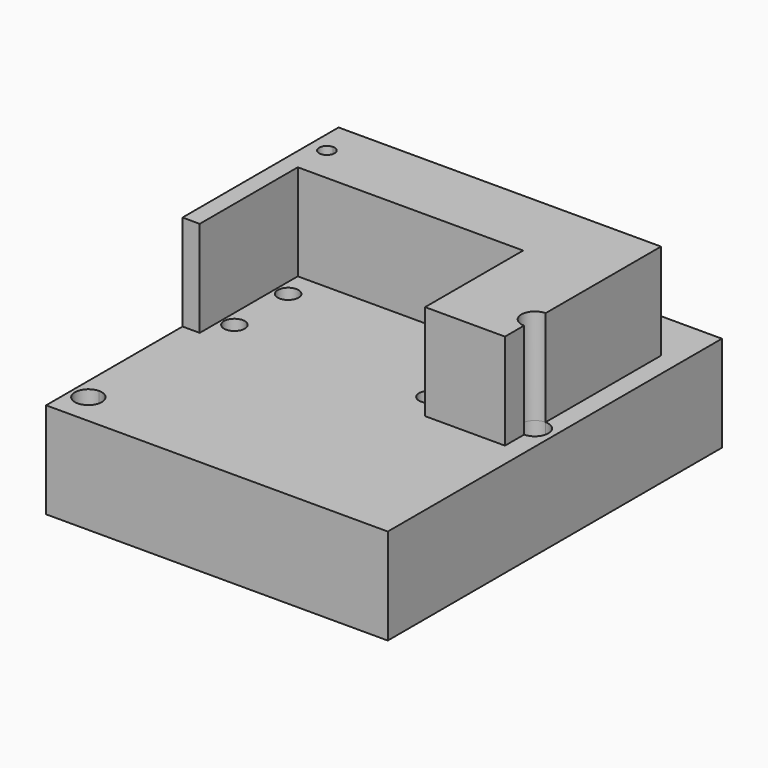
from build123d import *
from build123d import SkipClean  # not in build123d's __all__

# Parameters (mm, degrees)
F0_W     = 58.7
F0_H     = 31.916891567
F0_W_2   = 50.8
F0_H_2   = 17.5
F0_W_3   = 1.3
F0_H_3   = 0.083108433
F1_DEPTH = 25
F2_D     = 5.4102
F3_DEPTH = 25


with BuildPart() as f1:
    # F0 (on Top) → F1 (new body)
    with BuildSketch(Plane.XY):
        with BuildLine():
            ThreePointArc((0, 3.5), (2.4748737342, 2.4748737342), (3.5, 0))
            Line((3.5, 0), (79.5, 0))
            Line((79.5, 0), (79.5, 36.256108433))
            Line((79.5, 36.256108433), (58.7, 36.256108433))
            Line((58.7, 36.256108433), (58.7, 36.173))
            Line((58.7, 36.173), (0, 36.173))
            Line((0, 36.173), (0, 3.5))
        make_face()
        with BuildLine():
            Line((58.7, 36.256108433), (79.5, 36.256108433))
            Line((79.5, 36.256108433), (79.5, 42.475))
            ThreePointArc((79.5, 42.475), (76, 45.975), (79.5, 49.475))
            Line((79.5, 49.475), (79.5, 87.056108433))
            Line((79.5, 87.056108433), (0, 87.056108433))
            Line((0, 87.056108433), (0, 79.6536390185))
            ThreePointArc((0, 79.6536390185), (1.4142135624, 79.0678525809), (2, 77.6536390185))
            ThreePointArc((2, 77.6536390185), (1.4142135624, 76.2394254562), (0, 75.6536390185))
            Line((0, 75.6536390185), (0, 68.173))
            Line((0, 68.173), (58.7, 68.173))
            Line((58.7, 68.173), (58.7, 36.256108433))
        make_face()
        with Locations((29.35, 52.2145542165)):
            Rectangle(F0_W, F0_H)
        with Locations((28.7, 52.173)):
            Rectangle(F0_W_2, F0_H_2, mode=Mode.SUBTRACT)
        with BuildLine():
            Line((79.5, 0), (3.5, 0))
            ThreePointArc((3.5, 0), (-2.4748737342, -2.4748737342), (0, 3.5))
            Line((0, 3.5), (0, 36.173))
            Line((0, 36.173), (-1.3, 36.173))
            Line((-1.3, 36.173), (-1.3, 36.256108433))
            Line((-1.3, 36.256108433), (-4.48, 36.256108433))
            Line((-4.48, 36.256108433), (-4.48, -8.1671467051))
            Line((-4.48, -8.1671467051), (84.52, -8.1671467051))
            Line((84.52, -8.1671467051), (84.52, 36.256108433))
            Line((84.52, 36.256108433), (79.5, 36.256108433))
            Line((79.5, 36.256108433), (79.5, 0))
        make_face()
        with Locations((28.7, 52.173)):
            Rectangle(F0_W_2, F0_H_2)
        with BuildLine():
            Line((79.5, 87.056108433), (84.52, 87.056108433))
            Line((84.52, 87.056108433), (84.52, 100.6101816893))
            Line((84.52, 100.6101816893), (28.7, 100.6101816893))
            Line((28.7, 100.6101816893), (-4.48, 100.6101816893))
            Line((-4.48, 100.6101816893), (-4.48, 87.056108433))
            Line((-4.48, 87.056108433), (0, 87.056108433))
            Line((0, 87.056108433), (0, 88.45))
            ThreePointArc((0, 88.45), (-2.4748737342, 94.4248737342), (3.5, 91.95))
            Line((3.5, 91.95), (79.5, 91.95))
            Line((79.5, 91.95), (79.5, 87.056108433))
        make_face()
        with BuildLine():
            Line((0, 87.056108433), (79.5, 87.056108433))
            Line((79.5, 87.056108433), (79.5, 91.95))
            Line((79.5, 91.95), (3.5, 91.95))
            ThreePointArc((3.5, 91.95), (2.4748737342, 89.4751262658), (0, 88.45))
            Line((0, 88.45), (0, 87.056108433))
        make_face()
        with BuildLine():
            Line((79.5, 42.475), (79.5, 36.256108433))
            Line((79.5, 36.256108433), (84.52, 36.256108433))
            Line((84.52, 36.256108433), (84.52, 87.056108433))
            Line((84.52, 87.056108433), (79.5, 87.056108433))
            Line((79.5, 87.056108433), (79.5, 49.475))
            ThreePointArc((79.5, 49.475), (81.9748737342, 48.4498737342), (83, 45.975))
            ThreePointArc((83, 45.975), (81.9748737342, 43.5001262658), (79.5, 42.475))
        make_face()
        with BuildLine():
            Line((-1.3, 68.173), (0, 68.173))
            Line((0, 68.173), (0, 75.6536390185))
            ThreePointArc((0, 75.6536390185), (-2, 77.6536390185), (0, 79.6536390185))
            Line((0, 79.6536390185), (0, 87.056108433))
            Line((0, 87.056108433), (-4.48, 87.056108433))
            Line((-4.48, 87.056108433), (-4.48, 36.256108433))
            Line((-4.48, 36.256108433), (-1.3, 36.256108433))
            Line((-1.3, 36.256108433), (-1.3, 68.173))
        make_face()
        with Locations((-0.65, 52.2145542165)):
            Rectangle(F0_W_3, F0_H)
        with Locations((29.35, 36.2145542165)):
            Rectangle(F0_W, F0_H_3)
        with Locations((-0.65, 36.2145542165)):
            Rectangle(F0_W_3, F0_H_3)
    extrude(amount=-F1_DEPTH)

    # F2 (through all)
    with Locations(Plane.XY):
        with Locations((3.3, 60.923), (3.3, 43.423), (54.1, 43.423), (54.1, 60.923)):
            Hole(F2_D / 2)

    # F0 (on Top) → F3 (join)
    with BuildSketch(Plane.XY):
        with BuildLine():
            Line((-1.3, 68.173), (0, 68.173))
            Line((0, 68.173), (0, 75.6536390185))
            ThreePointArc((0, 75.6536390185), (-2, 77.6536390185), (0, 79.6536390185))
            Line((0, 79.6536390185), (0, 87.056108433))
            Line((0, 87.056108433), (-4.48, 87.056108433))
            Line((-4.48, 87.056108433), (-4.48, 36.256108433))
            Line((-4.48, 36.256108433), (-1.3, 36.256108433))
            Line((-1.3, 36.256108433), (-1.3, 68.173))
        make_face()
        with BuildLine():
            Line((58.7, 36.256108433), (79.5, 36.256108433))
            Line((79.5, 36.256108433), (79.5, 42.475))
            ThreePointArc((79.5, 42.475), (76, 45.975), (79.5, 49.475))
            Line((79.5, 49.475), (79.5, 87.056108433))
            Line((79.5, 87.056108433), (0, 87.056108433))
            Line((0, 87.056108433), (0, 79.6536390185))
            ThreePointArc((0, 79.6536390185), (1.4142135624, 79.0678525809), (2, 77.6536390185))
            ThreePointArc((2, 77.6536390185), (1.4142135624, 76.2394254562), (0, 75.6536390185))
            Line((0, 75.6536390185), (0, 68.173))
            Line((0, 68.173), (58.7, 68.173))
            Line((58.7, 68.173), (58.7, 36.256108433))
        make_face()
        with Locations((-0.65, 52.2145542165)):
            Rectangle(F0_W_3, F0_H)
    with SkipClean():  # cleaning this boolean's faces spoils the solid; the shape is the same uncleaned
        extrude(amount=F3_DEPTH)


solid = f1.part
